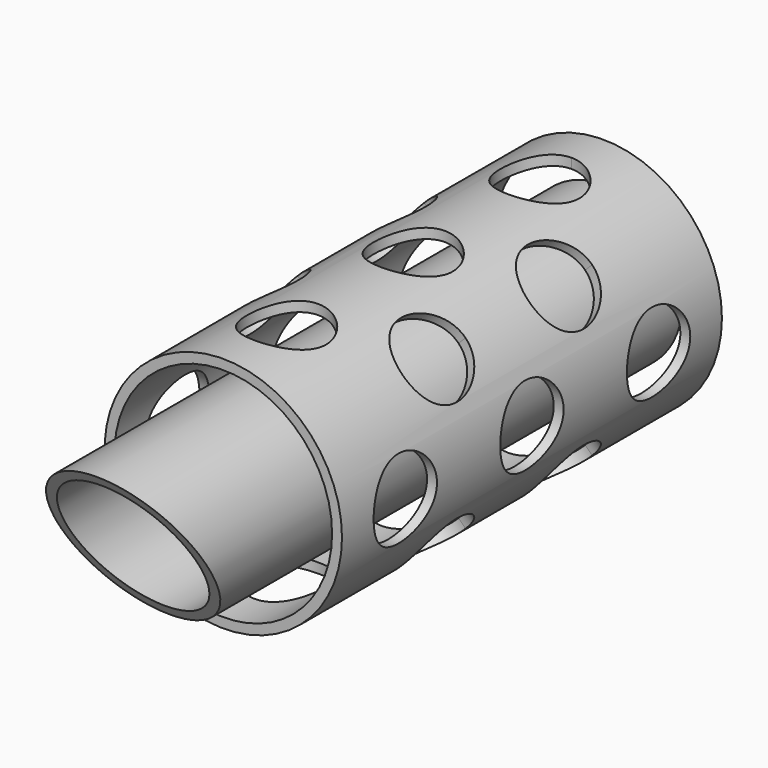
from build123d import *

# Parameters (mm, degrees)
F0_R      = 19.05
F0_R_2    = 17.4625
F1_DEPTH  = 76.2
F7_DEPTH  = 25.4
F2_R      = 6.35
F8_DEPTH  = 25.4
F9_DEPTH  = 25.4
F10_R     = 6.35
F11_DEPTH = 25.4
F0_R_3    = 12.7
F0_R_4    = 11.1125
F12_DEPTH = 101.6
F14_DEPTH = 12.7


with BuildPart() as f1:
    # F0 (on Front) → F1 (new body)
    with BuildSketch(Plane.XZ):
        Circle(F0_R)
        Circle(F0_R_2, mode=Mode.SUBTRACT)
    extrude(amount=F1_DEPTH)

    # F4 (on line) → F7 (cut, symmetric)
    with BuildSketch(Plane(origin=(0, 0, 0), x_dir=(0.7071067812, 0, 0.7071067812), z_dir=(0.7071067812, 0, -0.7071067812))):
        with BuildLine():
            ThreePointArc((0, 57.15), (-6.35, 50.8), (0, 44.45))
            Line((0, 44.45), (0, 57.15))
        make_face()
        with BuildLine():
            Line((0, 57.15), (0, 44.45))
            ThreePointArc((0, 44.45), (4.4901280605, 46.3098719395), (6.35, 50.8))
            ThreePointArc((6.35, 50.8), (4.4901280605, 55.2901280605), (0, 57.15))
        make_face()
        with BuildLine():
            ThreePointArc((6.35, 25.4), (4.4901280605, 29.8901280605), (0, 31.75))
            Line((0, 31.75), (0, 19.05))
            ThreePointArc((0, 19.05), (4.4901280605, 20.9098719395), (6.35, 25.4))
        make_face()
        with BuildLine():
            Line((0, 19.05), (0, 31.75))
            ThreePointArc((0, 31.75), (-6.35, 25.4), (0, 19.05))
        make_face()
    extrude(amount=F7_DEPTH, both=True, mode=Mode.SUBTRACT)

    # F2 (on Right) → F8 (cut, symmetric)
    with BuildSketch(Plane.YZ):
        with Locations((-63.5, 0)):
            Circle(F2_R)
        with BuildLine():
            Line((-38.1, 0), (-31.75, 0))
            ThreePointArc((-31.75, 0), (-38.1, 6.35), (-44.45, 0))
            Line((-44.45, 0), (-38.1, 0))
        make_face()
        with BuildLine():
            Line((-12.7, 0), (-6.35, 0))
            ThreePointArc((-6.35, 0), (-12.7, 6.35), (-19.05, 0))
            Line((-19.05, 0), (-12.7, 0))
        make_face()
        with BuildLine():
            ThreePointArc((-44.45, 0), (-38.1, -6.35), (-31.75, 0))
            Line((-31.75, 0), (-38.1, 0))
            Line((-38.1, 0), (-44.45, 0))
        make_face()
        with BuildLine():
            ThreePointArc((-19.05, 0), (-12.7, -6.35), (-6.35, 0))
            Line((-6.35, 0), (-12.7, 0))
            Line((-12.7, 0), (-19.05, 0))
        make_face()
    extrude(amount=F8_DEPTH, both=True, mode=Mode.SUBTRACT)

    # F6 (on line) → F9 (cut, symmetric)
    with BuildSketch(Plane(origin=(0, 0, 0), x_dir=(0.7071067812, 0, -0.7071067812), z_dir=(-0.7071067812, 0, -0.7071067812))):
        with BuildLine():
            ThreePointArc((0, 57.15), (-6.35, 50.8), (0, 44.45))
            Line((0, 44.45), (0, 57.15))
        make_face()
        with BuildLine():
            Line((0, 57.15), (0, 44.45))
            ThreePointArc((0, 44.45), (4.4901280605, 46.3098719395), (6.35, 50.8))
            ThreePointArc((6.35, 50.8), (4.4901280605, 55.2901280605), (0, 57.15))
        make_face()
        with BuildLine():
            ThreePointArc((6.35, 25.4), (4.4901280605, 29.8901280605), (0, 31.75))
            Line((0, 31.75), (0, 19.05))
            ThreePointArc((0, 19.05), (4.4901280605, 20.9098719395), (6.35, 25.4))
        make_face()
        with BuildLine():
            Line((0, 19.05), (0, 31.75))
            ThreePointArc((0, 31.75), (-6.35, 25.4), (0, 19.05))
        make_face()
    extrude(amount=F9_DEPTH, both=True, mode=Mode.SUBTRACT)

    # F10 (on Top) → F11 (cut, symmetric)
    with BuildSketch(Plane.XY):
        with BuildLine():
            ThreePointArc((0, -6.35), (-4.4901280605, -17.1901280605), (6.35, -12.7))
            ThreePointArc((6.35, -12.7), (4.4901280605, -8.2098719395), (0, -6.35))
        make_face()
        with Locations((0, -38.1)):
            Circle(F10_R)
        with Locations((0, -63.5)):
            Circle(F10_R)
    extrude(amount=F11_DEPTH, both=True, mode=Mode.SUBTRACT)


with BuildPart() as f12:
    # F0 (on Front) → F12 (new body)
    with BuildSketch(Plane.XZ):
        Circle(F0_R_3)
        Circle(F0_R_4, mode=Mode.SUBTRACT)
    extrude(amount=F12_DEPTH)

    # F13 (on Right) → F14 (cut, symmetric)
    with BuildSketch(Plane.YZ):
        Polygon((-101.6, 12.7), (-101.6, -12.7), (-86.9353031626, -12.7), align=None)
    extrude(amount=F14_DEPTH, both=True, mode=Mode.SUBTRACT)


solid = Compound([f1.part, f12.part])
